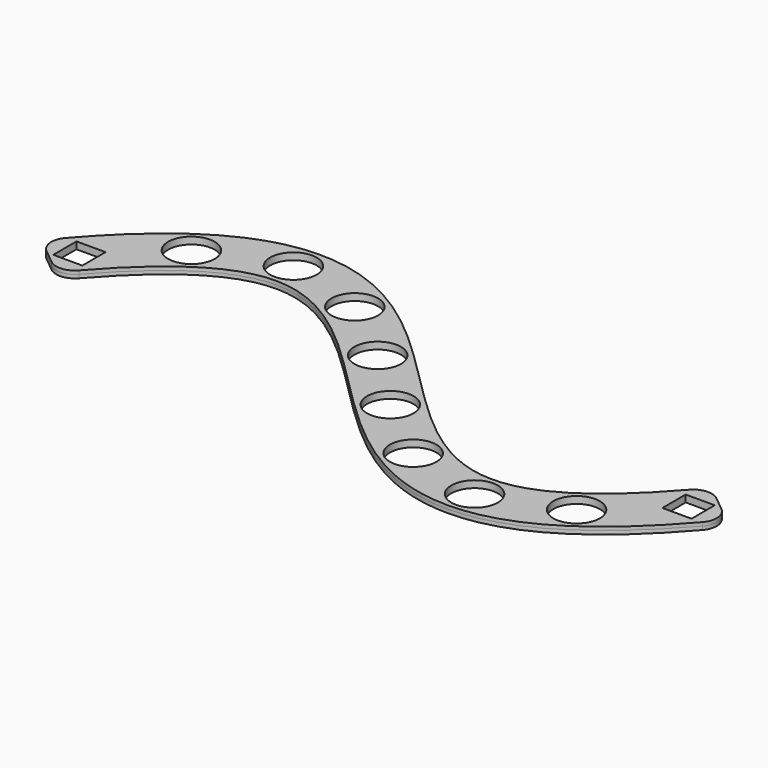
from build123d import *

# Parameters (mm, degrees)
F1_DEPTH = 4.7625
F2_R     = 25.4
F4_DEPTH = 9.5260001
F6_D     = 63.5


# Not quite as in the source:
# - the dataset's text gives a spline's control points without its knots; the knots are read off the source's solid


with BuildPart() as f1:
    # F0 (on Top) → F1 (new body, symmetric)
    with BuildSketch(Plane.XY):
        with BuildLine():
            Line((457.2, 0), (427.7135674749, 24.1279981959))
            add(Edge.make_bspline(
                [(427.7135674749, 24.1279981959), (415.401452544, 9.0815636262), (391.5568474097, -17.9663635403), (358.1835287083, -49.9592074326), (332.4481081466, -69.9872803487), (313.1509511046, -82.4055791393), (299.3257626721, -90.0286211782), (286.1389721031, -96.0801872695), (273.5625977918, -100.6881431755), (261.5453180986, -103.982234721), (250.0106264373, -106.0855995801), (238.8603469438, -107.1048358808), (227.9837906484, -107.1221107417), (217.2705806026, -106.1922117803), (206.6232898672, -104.3457680649), (195.9661581442, -101.5972112602), (185.2481705871, -97.9545266237), (174.4409831077, -93.4274516898), (159.8986837125, -86.2361090529), (141.4733808743, -75.144246862), (119.0424918671, -58.8059316541), (96.3698825334, -39.9001940342), (73.4896775508, -18.9497857472), (50.3874129932, 3.4950212864), (27.0040322071, 26.8770557427), (3.2410683575, 50.641365922), (-21.0374723931, 74.2379110716), (-46.0069940638, 97.118870063), (-71.8874934014, 118.7295223643), (-98.9475557558, 138.4876272681), (-122.7416318548, 152.871979952), (-142.6782176272, 162.7466318576), (-158.1111926165, 169.2234400955), (-174.0436737051, 174.6509018391), (-190.476624389, 178.9006305662), (-207.3883374056, 181.8424874779), (-224.7323600412, 183.3527801823), (-242.4405729405, 183.324013691), (-260.4319067391, 181.672851565), (-278.6249800514, 178.3433368664), (-296.9509245974, 173.3039436668), (-315.362541375, 166.5396855836), (-333.8378163285, 158.0421843849), (-352.3780754365, 147.8011817768), (-377.2117679175, 131.7966191529), (-408.5449022245, 107.3180516252), (-446.9362987821, 70.4330326515), (-473.2794438798, 40.51246005), (-486.6864325251, 24.1279981959)],
                knots=[0, 0, 0, 0, 0.03125, 0.0625, 0.09375, 0.109375, 0.125, 0.140625, 0.15625, 0.171875, 0.1875, 0.203125, 0.21875, 0.234375, 0.25, 0.265625, 0.28125, 0.296875, 0.3125, 0.34375, 0.375, 0.40625, 0.4375, 0.46875, 0.5, 0.53125, 0.5625, 0.59375, 0.625, 0.65625, 0.6875, 0.703125, 0.71875, 0.734375, 0.75, 0.765625, 0.78125, 0.796875, 0.8125, 0.828125, 0.84375, 0.859375, 0.875, 0.890625, 0.90625, 0.9375, 0.96875, 1, 1, 1, 1], degree=3))
            Line((-486.6864325251, 24.1279981959), (-457.2, 0))
            Line((-457.2, 0), (-427.7135674749, -24.1279981959))
            add(Edge.make_bspline(
                [(486.6864325251, -24.1279981959), (473.2794438798, -40.51246005), (446.9362987821, -70.4330326515), (408.5449022245, -107.3180516252), (377.2117679175, -131.7966191529), (352.3780754365, -147.8011817768), (333.8378163285, -158.0421843849), (315.362541375, -166.5396855836), (296.9509245974, -173.3039436668), (278.6249800514, -178.3433368664), (260.4319067391, -181.672851565), (242.4405729405, -183.324013691), (224.7323600412, -183.3527801823), (207.3883374056, -181.8424874779), (190.476624389, -178.9006305662), (174.0436737051, -174.6509018391), (158.1111926165, -169.2234400955), (142.6782176272, -162.7466318576), (122.7416318548, -152.871979952), (98.9475557558, -138.4876272681), (71.8874934014, -118.7295223643), (46.0069940638, -97.118870063), (21.0374723931, -74.2379110716), (-3.2410683575, -50.641365922), (-27.0040322071, -26.8770557427), (-50.3874129932, -3.4950212864), (-73.4896775508, 18.9497857472), (-96.3698825334, 39.9001940342), (-119.0424918671, 58.8059316541), (-141.4733808743, 75.144246862), (-159.8986837125, 86.2361090529), (-174.4409831077, 93.4274516898), (-185.2481705871, 97.9545266237), (-195.9661581442, 101.5972112602), (-206.6232898672, 104.3457680649), (-217.2705806026, 106.1922117803), (-227.9837906484, 107.1221107417), (-238.8603469438, 107.1048358808), (-250.0106264373, 106.0855995801), (-261.5453180986, 103.982234721), (-273.5625977918, 100.6881431755), (-286.1389721031, 96.0801872695), (-299.3257626721, 90.0286211782), (-313.1509511046, 82.4055791393), (-332.4481081466, 69.9872803487), (-358.1835287083, 49.9592074326), (-391.5568474097, 17.9663635403), (-415.401452544, -9.0815636262), (-427.7135674749, -24.1279981959)],
                knots=[0, 0, 0, 0, 0.03125, 0.0625, 0.09375, 0.109375, 0.125, 0.140625, 0.15625, 0.171875, 0.1875, 0.203125, 0.21875, 0.234375, 0.25, 0.265625, 0.28125, 0.296875, 0.3125, 0.34375, 0.375, 0.40625, 0.4375, 0.46875, 0.5, 0.53125, 0.5625, 0.59375, 0.625, 0.65625, 0.6875, 0.703125, 0.71875, 0.734375, 0.75, 0.765625, 0.78125, 0.796875, 0.8125, 0.828125, 0.84375, 0.859375, 0.875, 0.890625, 0.90625, 0.9375, 0.96875, 1, 1, 1, 1], degree=3))
            Line((486.6864325251, -24.1279981959), (457.2, 0))
        make_face()
    extrude(amount=F1_DEPTH, both=True)

    # F2
    f2_edges = [f1.edges().sort_by_distance(p)[0] for p in [
        (-427.713567, -24.127998, -2.38125),
        (-427.713567, -24.127998, 2.38125),
        (-486.686433, 24.127998, -2.38125),
        (-486.686433, 24.127998, 2.38125),
        (486.686433, -24.127998, -2.38125),
        (486.686433, -24.127998, 2.38125),
        (427.713567, 24.127998, -2.38125),
        (427.713567, 24.127998, 2.38125),
    ]]
    fillet(f2_edges, radius=F2_R)

    # F3 (on face) → F4 (cut, through all)
    with BuildSketch(Plane.XY.offset(4.7625)):
        Polygon((-416.1504382002, 5.474325054), (-416.1504382002, 45.161825054), (-455.8379382002, 45.161825054), (-455.8379382002, 5.474325054), (-452.2318244009, 5.474325054), align=None)
        Polygon((455.8379382002, -45.1618250541), (455.8379382002, -5.4743250541), (452.2318244009, -5.4743250541), (416.1504382002, -5.4743250541), (416.1504382002, -45.1618250541), align=None)
    extrude(amount=-F4_DEPTH, mode=Mode.SUBTRACT)

    # F6 (through all)
    with Locations(Plane.XY.offset(4.7625)):
        with Locations((-347.2911395284, 105.5736822785), (-239.6882469243, 145.0400179253), (-129.807601036, 112.4483348558), (-40.8079355271, 40.2331447262), (40.8079355271, -40.2331447262), (129.807601036, -112.4483348558), (239.6882469243, -145.0400179253), (347.2911395284, -105.5736822785)):
            Hole(F6_D / 2)


solid = f1.part
